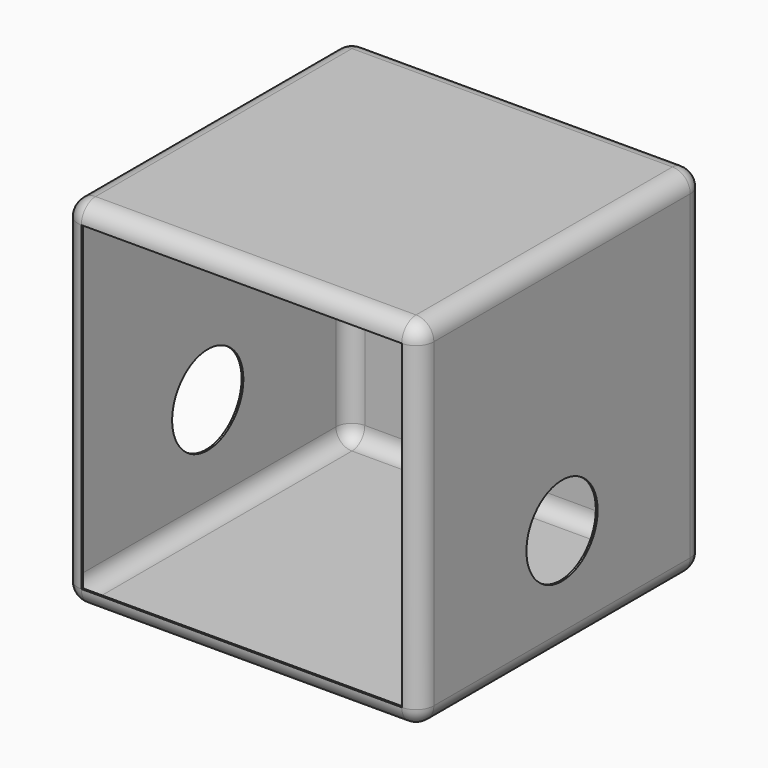
from build123d import *

# Parameters (mm, degrees)
F0_W     = 1000
F0_H     = 1000
F1_DEPTH = 1000
F2_R     = 50
F3_T     = -5
F4_R     = 125
F5_DEPTH = 650


# Not quite as in the source:
# - a shell that OpenCascade refuses in one call is made with other operations: the cavity is built on its own and cut out


with BuildPart() as f1:
    # F0 (on Top) → F1 (new body)
    with BuildSketch(Plane.XY):
        Rectangle(F0_W, F0_H)
    extrude(amount=F1_DEPTH)

    # F2
    f2_edges = [f1.edges().sort_by_distance(p)[0] for p in [
        (0, 500, 1000),
        (-500, 500, 500),
        (-500, 0, 1000),
        (500, 0, 1000),
        (500, 500, 500),
        (0, -500, 1000),
        (-500, -500, 500),
        (500, -500, 500),
        (500, 0, 0),
        (0, -500, 0),
        (0, 500, 0),
        (-500, 0, 0),
    ]]
    fillet(f2_edges, radius=F2_R)

    # F3: a shell. OpenCascade refuses it in one call, so the cavity is built on its own and cut out:
    # the body offset inwards by the wall thickness, plus a prism from it out through each open face.
    f3_core = offset(f1.part, amount=F3_T, mode=Mode.PRIVATE)
    f3_exits = [f3_core.faces().sort_by_distance(p)[0] for p in [
        (0, -495, 500),
    ]]
    add(f3_core, mode=Mode.SUBTRACT)
    extrude(f3_exits, amount=-F3_T, mode=Mode.SUBTRACT)

    # F4 (on Right) → F5 (cut, symmetric)
    with BuildSketch(Plane.YZ):
        with Locations((0, 300)):
            Circle(F4_R)
    extrude(amount=F5_DEPTH, both=True, mode=Mode.SUBTRACT)


solid = f1.part
